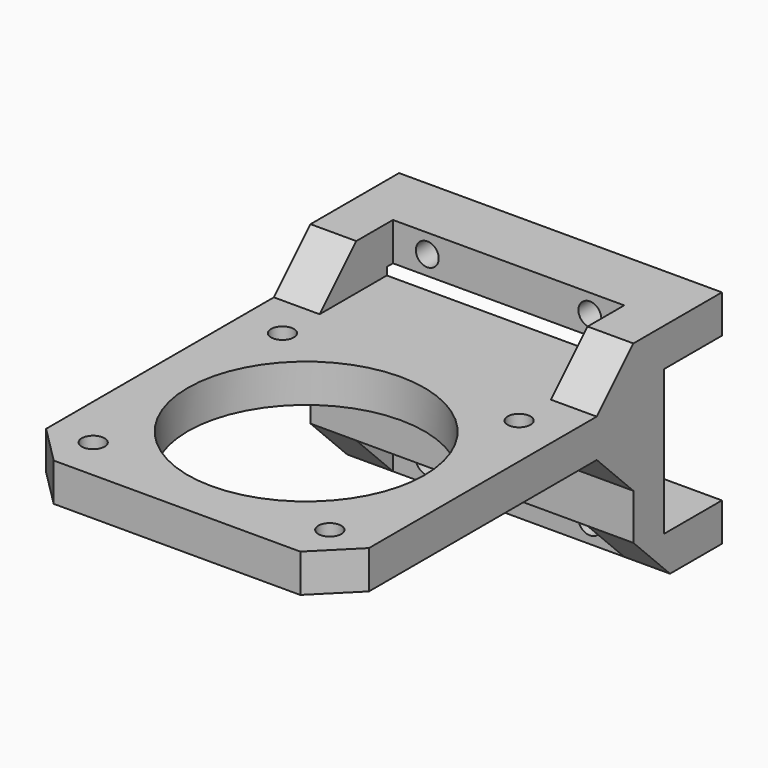
from build123d import *

# Parameters (mm, degrees)
F1_DEPTH  = 42.3
F3_W      = 30.3
F3_H      = 6
F4_DEPTH  = 6
F2_W      = 30.3
F2_H      = 6
F5_DEPTH  = 12
F6_SIZE   = 5.99999
F7_R      = 1.5
F8_DEPTH  = 8.501
F9_R      = 1.5
F10_DEPTH = 8.501
F11_R     = 1.5
F11_R_2   = 15.5
F12_DEPTH = 5
F13_SIZE  = 5


# Not quite as in the source:
# - a fillet or chamfer is up to 0.001 mm smaller than in the source, because OpenCascade refuses the exact size
# - a feature names something its author has since deleted; it is built from what else it names


with BuildPart() as f1:
    # F0 (on Right) → F1 (new body)
    with BuildSketch(Plane.YZ):
        Polygon((-9.5, 9.5), (0, 9.5), (0, 14.5), (-14.5, 14.5), (-20.5, 14.5), (-20.5, 8.5), (-62.8, 8.5), (-62.8, 3.5), (-20.5, 3.5), (-20.5, -2.5), (-14.5, -2.5), (-14.5, -14.5), (0, -14.5), (0, -9.5), (-9.5, -9.5), align=None)
    extrude(amount=F1_DEPTH)

    # F3 (on face) → F4 (cut)
    with BuildSketch(Plane.XZ.offset(14.5)):
        with Locations((21.15, -11.5)):
            Rectangle(F3_W, F3_H)
    extrude(amount=-F4_DEPTH, mode=Mode.SUBTRACT)

    # F2 (on face) → F5 (cut)
    with BuildSketch(Plane.XZ.offset(20.5)):
        with Locations((21.15, 11.5)):
            Rectangle(F2_W, F2_H)
    extrude(amount=-F5_DEPTH, mode=Mode.SUBTRACT)

    # F6 (size 6 in the source; OpenCascade refuses exactly that, so slightly less here)
    f6_edges = [f1.edges().sort_by_distance(p)[0] for p in [
        (3, -14.5, -14.5),
        (39.3, -14.5, -14.5),
        (3, -20.5, 14.5),
        (39.3, -20.5, 14.5),
        (21.15, -20.5, -2.5),
    ]]
    chamfer(f6_edges, length=F6_SIZE)

    # F7 (on face) → F8 (cut, through all)
    with BuildSketch(Plane.XZ.offset(8.5)):
        with Locations((10.5, 12)):
            Circle(F7_R)
        with Locations((31.8, 12)):
            Circle(F7_R)
    extrude(amount=-F8_DEPTH, mode=Mode.SUBTRACT)

    # F9 (on face) → F10 (cut, through all)
    with BuildSketch(Plane.XZ.offset(8.5)):
        with Locations((10.5, -12)):
            Circle(F9_R)
        with Locations((31.8, -12)):
            Circle(F9_R)
    extrude(amount=-F10_DEPTH, mode=Mode.SUBTRACT)

    # F11 (on face) → F12 (cut, through all)
    with BuildSketch(Plane.XY.offset(8.5)):
        with Locations((5.65, -57.15)):
            Circle(F11_R)
        with Locations((5.65, -26.15)):
            Circle(F11_R)
        with Locations((36.65, -26.15)):
            Circle(F11_R)
        with Locations((36.65, -57.15)):
            Circle(F11_R)
        with Locations((21.15, -41.65)):
            Circle(F11_R_2)
    extrude(amount=-F12_DEPTH, mode=Mode.SUBTRACT)

    # F13
    f13_edges = [f1.edges().sort_by_distance(p)[0] for p in [
        (42.3, -62.8, 6),
        (0, -62.8, 6),
    ]]
    chamfer(f13_edges, length=F13_SIZE)


solid = f1.part
